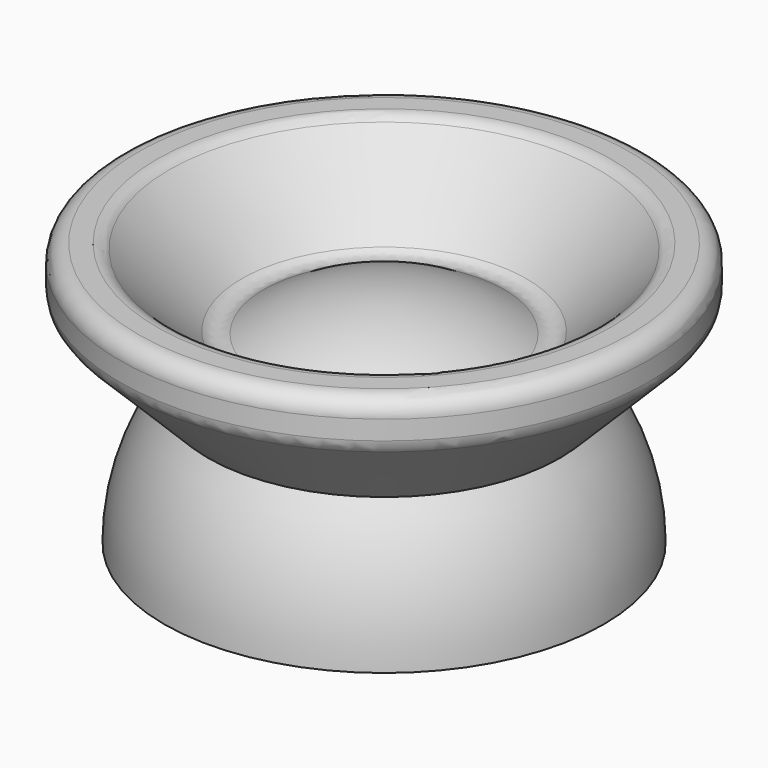
from build123d import *

# Parameters (mm, degrees)
F2_R = 5.08


with BuildPart() as f1:
    # F0 (on Front) → F1 (revolve)
    with BuildSketch(Plane.XZ):
        with BuildLine():
            Line((0, 0), (63.5, 0))
            ThreePointArc((63.5, 0), (60.2413894262, 20.0804631421), (50.8, 38.1))
            ThreePointArc((50.8, 38.1), (44.9012806053, 44.9012806053), (38.1, 50.8))
            ThreePointArc((38.1, 50.8), (20.0804631421, 60.2413894262), (0, 63.5))
            Line((0, 63.5), (0, 0))
        make_face()
        with BuildLine():
            ThreePointArc((38.1, 50.8), (44.9012806053, 44.9012806053), (50.8, 38.1))
            Line((50.8, 38.1), (76.2, 63.5))
            Line((76.2, 63.5), (76.2, 76.2))
            Line((76.2, 76.2), (63.5, 76.2))
            Line((63.5, 76.2), (38.1, 50.8))
        make_face()
    revolve(axis=Axis((0, 0, -31.75), (0, 0, -1)))

    # F2
    f2_edges = [f1.edges().sort_by_distance(p)[0] for p in [
        (-63.5, 0, 76.2),
        (-76.2, 0, 76.2),
        (-76.2, 0, 63.5),
        (-38.1, 0, 50.8),
    ]]
    fillet(f2_edges, radius=F2_R)


solid = f1.part
